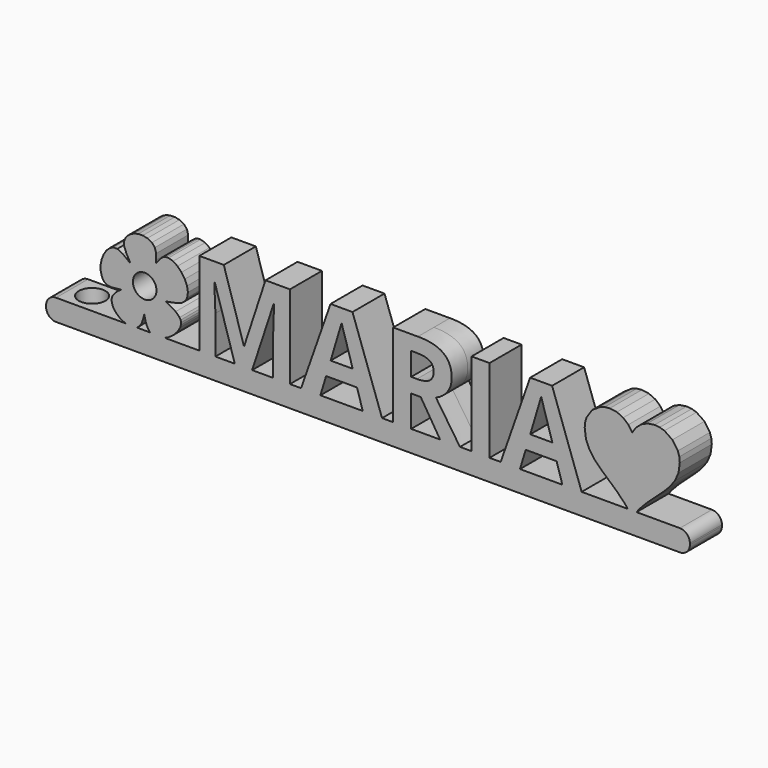
from build123d import *

# Parameters (mm, degrees)
F0_R         = 1.7660260944
F0_TEXT_SIZE = 17.7951454122
F1_DEPTH     = 3
F2_W         = 89
F2_H         = 6
F3_DEPTH     = 0.2
F4_DEPTH     = 3
F5_W         = 6
F5_H         = 3.2
F6_DEPTH     = 7.5
F7_R         = 1.5
F8_R         = 2
F9_DEPTH     = 4
F10_R        = 1.5


# Not quite as in the source:
# - Text() gives the source's letters only with a copy of the font that has no kerning and outlines rounded to 1/6400 em; it was checked with that copy


with BuildPart() as f1:
    # F0 (on Front) → F1 (new body, symmetric)
    with BuildSketch(Plane.XZ):
        Polygon((-9.8962181259, -0.0299609487), (-9.3093152472, 0.0995427735), (-8.5310452338, 0.4643787281), (-7.7886221935, 1.0156229815), (-7.1753136859, 1.6703047867), (-6.7844076966, 2.345448762), (-6.6844409889, 2.697736103), (-6.6652413988, 3.0240118702), (-6.7312263226, 3.3305926174), (-6.8868132072, 3.6238062576), (-7.4844896445, 4.1953846804), (-8.4936258745, 4.789299945), (-8.9274018823, 5.0567831788), (-8.4181052429, 5.1580766137), (-7.3131137554, 5.3695361907), (-6.5480905692, 5.6521941874), (-6.0523445823, 6.043851435), (-5.7552051187, 6.5823041299), (-5.6420905942, 7.3346827833), (-5.7751165223, 8.1369112107), (-6.1089634595, 8.9328581362), (-6.5983028952, 9.6663968681), (-7.1978267956, 10.281407439), (-7.8622157172, 10.7217585729), (-8.546147975, 10.9313258196), (-8.8812811082, 10.9320270148), (-9.2043064176, 10.8539824368), (-9.6469000392, 10.5612860557), (-10.1400767255, 9.9810366231), (-10.4508130024, 9.5801644376), (-10.4068223535, 10.0271686751), (-10.3916193646, 10.9311557532), (-10.598433195, 11.6324207168), (-11.0363252865, 12.1480644274), (-11.7143548393, 12.4951945719), (-12.3982545289, 12.6383143795), (-13.0712303381, 12.6247535348), (-13.7032208938, 12.4733707309), (-14.2641853, 12.2030313855), (-14.7240621838, 11.8325941916), (-15.0528129411, 11.3809291004), (-15.2203761991, 10.8668948051), (-15.1967042361, 10.3093544817), (-14.8286469794, 9.4077545862), (-14.3529716358, 8.5454741101), (-14.2906102139, 8.4004774316), (-14.4811582303, 8.5293860258), (-15.3946726039, 9.2300894295), (-16.21802192, 9.6332437342), (-16.8030362894, 9.634121823), (-17.3568401554, 9.3699870508), (-17.8525159958, 8.8932532172), (-18.2631576982, 8.2563454299), (-18.5618432066, 7.5116797807), (-18.7216618753, 6.7116836696), (-18.7156984739, 5.9087754295), (-18.5170445979, 5.1553756349), (-18.2008868091, 4.6439944488), (-17.7512302174, 4.3560670179), (-17.1086136552, 4.2712956407), (-16.2135760559, 4.3694053341), (-15.7044514474, 4.4302814773), (-15.6696932647, 4.4000047008), (-15.7790195709, 4.3290260096), (-16.1651405309, 4.0708069691), (-16.5523139664, 3.7127982689), (-16.8671052824, 3.3322639471), (-17.0360798838, 3.0064680418), (-17.0831036318, 2.6043628391), (-17.0239245605, 2.1921008316), (-16.867618816, 1.7819255621), (-16.6232807801, 1.3860941234), (-16.3000002503, 1.0168545414), (-15.9068693162, 0.6864593752), (-15.4529754831, 0.4071521172), (-14.9474063577, 0.1911989779), (-14.4397479673, 0.0570083052), (-13.9840845603, 0.0188926715), (-13.5797273957, 0.0772799851), (-13.2259605822, 0.2326232662), (-12.9220907946, 0.485341356), (-12.6674066752, 0.8358849825), (-12.4612081239, 1.2846821047), (-12.3027905578, 1.8321743328), (-12.1879723822, 2.2557758958), (-12.1309056827, 2.0998483864), (-12.0112204133, 1.5291342486), (-11.8237778137, 0.9902805659), (-11.5954117235, 0.5466869075), (-11.3529559319, 0.2617414835), (-10.9521058183, 0.053843468), (-10.4551700276, -0.0442881949), align=None)
        with Locations((-12.1185852993, 6.0541479067)):
            Circle(F0_R, mode=Mode.SUBTRACT)
        Polygon((58.6602663837, 12.4433699982), (57.5992463837, 12.5970599982), (56.8406363837, 12.5204799982), (56.1338363837, 12.3008699982), (54.9364963837, 11.4933499982), (54.1288763837, 10.2961199982), (53.9092263837, 9.5893599982), (53.8326363837, 8.8307599982), (54.0211563837, 7.3860999982), (54.5418963837, 6.1597099982), (55.3276463837, 5.0814099982), (56.3111763837, 4.0810299982), (58.6080263837, 2.0250499982), (59.7926163837, 0.8247399982), (60.9156063837, -0.5860800018), (60.9598863837, -0.6500000018), (61.0029163837, -0.5851400018), (62.0808263837, 0.8234499982), (63.2441263837, 2.0333299982), (65.5477963837, 4.1212499982), (66.5485863837, 5.1327499982), (67.3535863837, 6.2116199982), (67.8899763837, 7.4226699982), (68.0849563837, 8.8307599982), (68.0083763837, 9.5893599982), (67.7887663837, 10.2961199982), (66.9812463837, 11.4933499982), (65.7840163837, 12.3008699982), (65.0772463837, 12.5204799982), (64.3186563837, 12.5970599982), (63.2576363837, 12.4433699982), (62.3165663837, 12.0123599982), (61.5366163837, 11.3491699982), (60.9589463837, 10.4989199982), (60.3812863837, 11.3491699982), (59.6013363837, 12.0123599982), align=None)
        with Locations((-5.5281280529, 0)):
            Text('MARIA', F0_TEXT_SIZE, font='Open Sans', font_style=FontStyle.BOLD, text_align=(TextAlign.LEFT, TextAlign.BOTTOM))
    extrude(amount=F1_DEPTH, both=True)



with BuildPart() as f3:
    # F2 (on Top) → F3 (new body)
    with BuildSketch(Plane.XY):
        with Locations((25.1, 0)):
            Rectangle(F2_W, F2_H)
    extrude(amount=F3_DEPTH)


with BuildPart() as f4:
    # F4 (new): a face of the model
    f4_faces = [f3.part.faces().sort_by_distance(p)[0] for p in [
        (25.1, 0, 0),
    ]]
    extrude(f4_faces, amount=F4_DEPTH)


with BuildPart() as f1_1:
    add(f1.part)

    add(f3.part)  # F6 merges F3

    add(f4.part)  # F6 merges F4
    # F5 (on face) → F6 (join)
    with BuildSketch(Plane(origin=(-19.4, 0, 0), x_dir=(0, -1, 0), z_dir=(-1, 0, 0))):
        with Locations((0, -1.4)):
            Rectangle(F5_W, F5_H)
    extrude(amount=F6_DEPTH)

    # F7
    f7_edges = [f1_1.edges().sort_by_distance(p)[0] for p in [
        (-26.9, 0, -3),
        (-26.9, 0, 0.2),
        (69.6, 0, -3),
    ]]
    fillet(f7_edges, radius=F7_R)

    # F8 (on face) → F9 (cut)
    with BuildSketch(Plane.XY.offset(0.2)):
        with Locations((-22.4, 0)):
            Circle(F8_R)
    extrude(amount=-F9_DEPTH, mode=Mode.SUBTRACT)

    # F10
    f10_edges = [f1_1.edges().sort_by_distance(p)[0] for p in [
        (69.6, 0, 0.2),
    ]]
    fillet(f10_edges, radius=F10_R)


solid = f1_1.part
